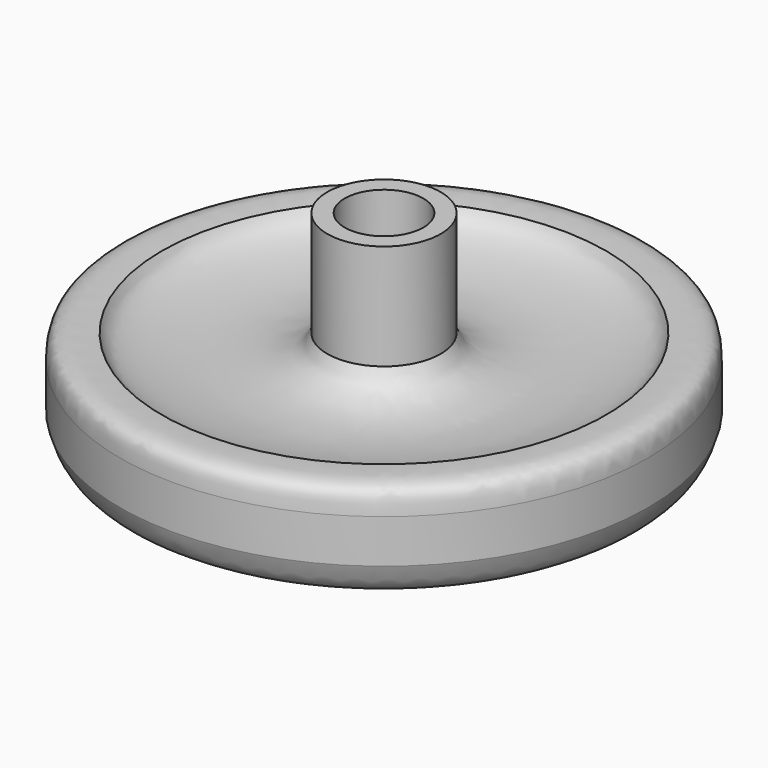
from build123d import *

# Parameters (mm, degrees)
F2_DEPTH = 12.7
F3_R     = 1.6348042273
F4_DEPTH = 19.6596
F5_R     = 4.7343922938
F6_DEPTH = 9.525


# Not quite as in the source:
# - a feature names something its author has since deleted; it is built from what else it names


with BuildPart() as f1:
    # F0 (on Front) → F1 (revolve)
    with BuildSketch(Plane.XZ):
        Polygon((0, 4.4785123318), (0, 8.1742972476), (-4.7625, 8.1742972476), (-6.8253115751, 8.1742972476), (-6.8253115751, 4.4785123318), align=None)
        with BuildLine():
            Line((0, 0), (0, 4.4785123318))
            Line((0, 4.4785123318), (-6.8253115751, 4.4785123318))
            Line((-6.8253115751, 4.4785123318), (-26.7162192613, 4.4785123318))
            Line((-26.7162192613, 4.4785123318), (-26.7162192613, 8.1742972476))
            add(Edge.make_bspline(
                [(-26.7162192613, 8.1742972476), (-28.491194666, 8.3112325103), (-31.642316511, 8.5543343001), (-31.7172676235, 6.2491747733), (-31.75, 5.2424739115)],
                knots=[0, 0, 0, 0, 0.5632836469, 1, 1, 1, 1], degree=3))
            Line((-31.75, 5.2424739115), (-31.75, 0))
            Line((-31.75, 0), (0, 0))
        make_face()
        with BuildLine():
            Line((0, -4.1164574213), (0, 0))
            Line((0, 0), (-31.75, 0))
            add(Edge.make_bspline(
                [(-31.75, 0), (-31.4027760977, -1.1805231122), (-30.8776022636, -2.9683987357), (-28.8835885285, -3.872962504), (-28.1014181098, -4.1164574213)],
                knots=[0, 0, 0, 0, 0.4216161755, 0.638071699, 0.638071699, 0.638071699, 0.638071699], degree=3))
            Line((-28.1014181098, -4.1164574213), (0, -4.1164574213))
        make_face()
        with BuildLine():
            Line((-26.7162192613, 4.4785123318), (-6.8253115751, 4.4785123318))
            Line((-6.8253115751, 4.4785123318), (-6.8253115751, 8.1742972476))
            add(Edge.make_bspline(
                [(-26.7162192613, 8.1742972476), (-26.6031223158, 7.9651163147), (-26.3129395448, 7.4284024145), (-24.8626402231, 5.7951518451), (-14.4096521607, 4.0441326554), (-7.9711337562, 5.8305330049), (-7.1335011103, 7.5438995955), (-6.8253115751, 8.1742972476)],
                knots=[0, 0, 0, 0, 0.0911428309, 0.23385317, 0.5753642763, 0.8437641047, 1, 1, 1, 1], degree=3))
            Line((-26.7162192613, 8.1742972476), (-26.7162192613, 4.4785123318))
        make_face()
        with BuildLine():
            Line((0, -17.5582827176), (0, -4.1164574213))
            Line((0, -4.1164574213), (-28.1014181098, -4.1164574213))
            add(Edge.make_bspline(
                [(-28.1014181098, -4.1164574213), (-26.8429354447, -4.3749563957), (-25.5844527797, -4.6334553702), (-23.5869744443, -4.9854039485)],
                knots=[0, 0, 0, 0, 0.1942754447, 0.1942754447, 0.1942754447, 0.1942754447], degree=3))
            add(Edge.make_bspline(
                [(-23.5869744443, -4.9854039485), (-20.1583969161, -5.5895071147), (-9.8833890293, -7.2014232525), (-3.0789336633, -13.7945227485), (-0.8981879892, -16.4603168735), (0, -17.5582827176)],
                knots=[0.1942754447, 0.1942754447, 0.1942754447, 0.1942754447, 0.5277400996, 0.8054893905, 1, 1, 1, 1], degree=3))
        make_face()
        with BuildLine():
            add(Edge.make_bspline(
                [(-28.1014181098, -4.1164574213), (-26.8429354447, -4.3749563957), (-25.5844527797, -4.6334553702), (-23.5869744443, -4.9854039485)],
                knots=[0, 0, 0, 0, 0.1942754447, 0.1942754447, 0.1942754447, 0.1942754447], degree=3))
            add(Edge.make_bspline(
                [(-28.1014181098, -4.1164574213), (-26.7935761747, -4.5235974207), (-25.1901235467, -4.7535844093), (-23.5869744443, -4.9854039485)],
                knots=[0.638071699, 0.638071699, 0.638071699, 0.638071699, 1, 1, 1, 1], degree=3))
        make_face()
    revolve(axis=Axis((0, 0, -2.0582287107), (0, 0, 1)))

    # F2 (add): a face of the model
    f2_faces = [f1.faces().sort_by_distance(p)[0] for p in [
        (0, 0, 8.1742972476),
    ]]
    extrude(f2_faces, amount=F2_DEPTH)

    # F3 (on Top) → F4 (cut)
    with BuildSketch(Plane.XY):
        Circle(F3_R)
    extrude(amount=-F4_DEPTH, mode=Mode.SUBTRACT)

    # F5 (on face) → F6 (cut)
    with BuildSketch(Plane.XY.offset(20.8742972476)):
        Circle(F5_R)
    extrude(amount=-F6_DEPTH, mode=Mode.SUBTRACT)


solid = f1.part
